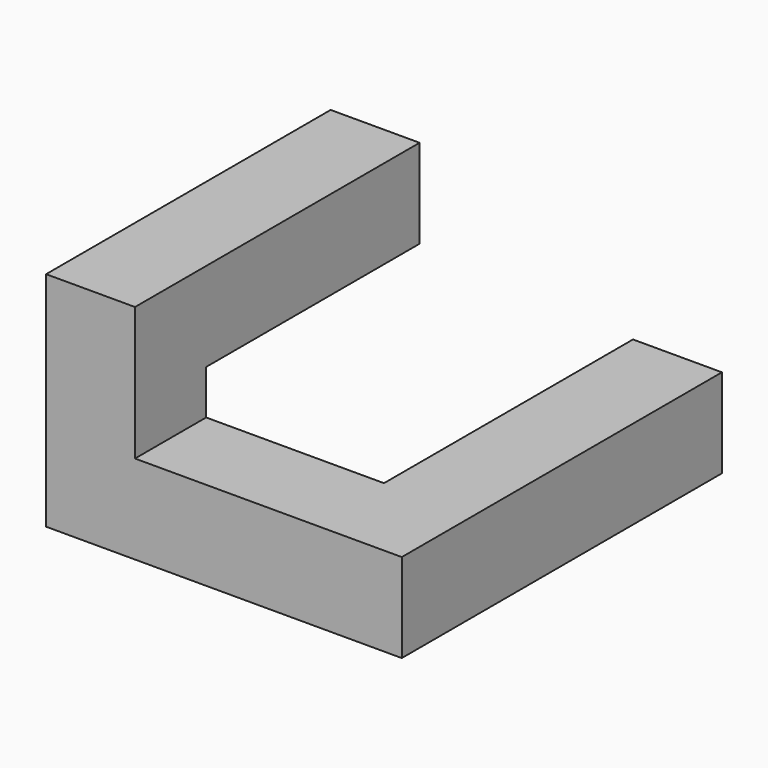
from build123d import *

# Parameters (mm, degrees)
F4_DEPTH = 25.4
F5_W     = 25.4
F5_H     = 25.4
F6_DEPTH = 76.2
F7_W     = 25.4
F7_H     = 25.4
F8_DEPTH = 88.9


# Not quite as in the source:
# - a variable given as a bare number and used for a length is read in inches; the dataset says mm whatever the document's units were


with BuildPart() as f4:
    # F3 (on Front) → F4 (new body)
    with BuildSketch(Plane.XZ):
        Polygon((0, 25.4), (0, 0), (25.4, 0), (101.6, 0), (101.6, 25.4), (25.4, 25.4), (25.4, 63.5), (0, 63.5), align=None)
    extrude(amount=-F4_DEPTH)

    # F5 (on face) → F6 (join)
    with BuildSketch(Plane(origin=(0, 25.4, 0), x_dir=(-1, 0, 0), z_dir=(0, 1, 0))):
        with Locations((-12.7, 50.8)):
            Rectangle(F5_W, F5_H)
    extrude(amount=F6_DEPTH)

    # F7 (on face) → F8 (join)
    with BuildSketch(Plane(origin=(0, 25.4, 0), x_dir=(-1, 0, 0), z_dir=(0, 1, 0))):
        with Locations((-88.9, 12.7)):
            Rectangle(F7_W, F7_H)
    extrude(amount=F8_DEPTH)


solid = f4.part
